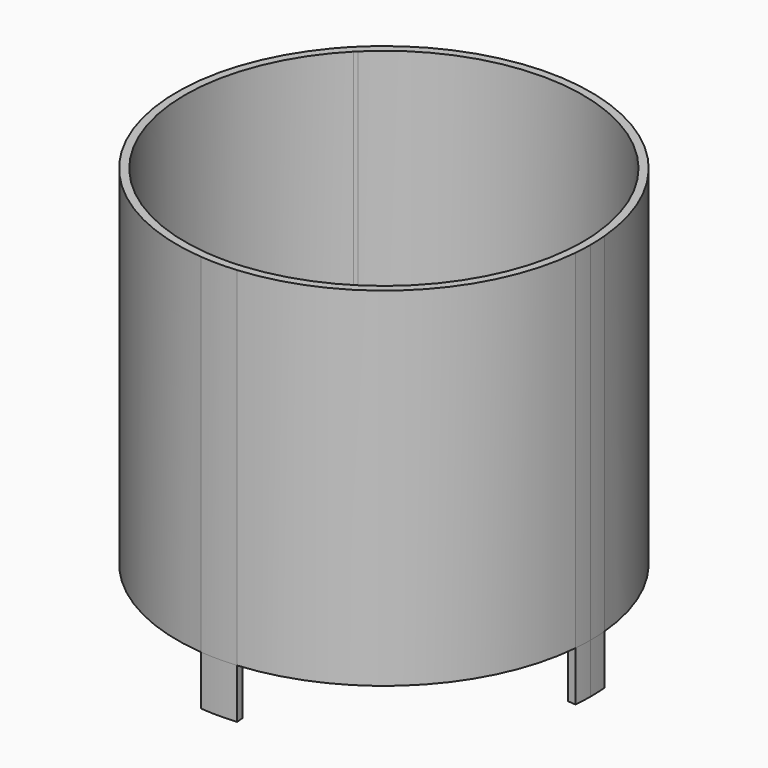
from build123d import *

# Parameters (mm, degrees)
F1_DEPTH = 80
F2_DEPTH = 70


with BuildPart() as f1:
    # F0 (on Top) → F1 (new body)
    with BuildSketch(Plane.XY):
        with BuildLine():
            Line((-70.6127849928, 75.5430583301), (-71.6412451683, 76.7687294391))
            ThreePointArc((-71.6412451683, 76.7687294391), (-74.3169227027, 74.3169227027), (-76.7687294391, 71.6412451683))
            Line((-76.7687294391, 71.6412451683), (-75.5430583301, 70.6127849928))
            ThreePointArc((-75.5430583301, 70.6127849928), (-73.1855518528, 73.1855518528), (-70.6127849928, 75.5430583301))
        make_face()
    extrude(amount=-F1_DEPTH)


with BuildPart() as f1b:
    # F0 (on Top) → F1, piece 2 (new body)
    with BuildSketch(Plane.XY):
        with BuildLine():
            Line((-5.0534926817, 41.4150508954), (-3.4595811647, 41.275601707))
            ThreePointArc((-3.4595811647, 41.275601707), (-3.3408745875, 43.0867140909), (-3.3012806053, 44.9012806053))
            ThreePointArc((-3.3012806053, 44.9012806053), (-3.3408745875, 46.7158471197), (-3.4595811647, 48.5269595036))
            Line((-3.4595811647, 48.5269595036), (-5.0534926817, 48.3875103153))
            ThreePointArc((-5.0534926817, 48.3875103153), (-4.9393517421, 46.6460561), (-4.9012806053, 44.9012806053))
            ThreePointArc((-4.9012806053, 44.9012806053), (-4.9393517421, 43.1565051107), (-5.0534926817, 41.4150508954))
        make_face()
    extrude(amount=-F1_DEPTH)


with BuildPart() as f1c:
    # F0 (on Top) → F1, piece 3 (new body)
    with BuildSketch(Plane.XY):
        with BuildLine():
            ThreePointArc((-48.5269595036, 3.4595811647), (-44.9012806053, 3.3012806053), (-41.275601707, 3.4595811647))
            Line((-41.275601707, 3.4595811647), (-41.4150508954, 5.0534926817))
            ThreePointArc((-41.4150508954, 5.0534926817), (-44.9012806053, 4.9012806053), (-48.3875103153, 5.0534926817))
            Line((-48.3875103153, 5.0534926817), (-48.5269595036, 3.4595811647))
        make_face()
    extrude(amount=-F1_DEPTH)


with BuildPart() as f2:
    # F0 (on Top) → F2 (new body)
    with BuildSketch(Plane.XY):
        with BuildLine():
            Line((-5.0534926817, 48.3875103153), (-3.4595811647, 48.5269595036))
            ThreePointArc((-3.4595811647, 48.5269595036), (-28.981649819, 83.3346691578), (-71.6412451683, 76.7687294391))
            Line((-71.6412451683, 76.7687294391), (-70.6127849928, 75.5430583301))
            ThreePointArc((-70.6127849928, 75.5430583301), (-29.5939433107, 81.8564619058), (-5.0534926817, 48.3875103153))
        make_face()
        with BuildLine():
            Line((-70.6127849928, 75.5430583301), (-71.6412451683, 76.7687294391))
            ThreePointArc((-71.6412451683, 76.7687294391), (-74.3169227027, 74.3169227027), (-76.7687294391, 71.6412451683))
            Line((-76.7687294391, 71.6412451683), (-75.5430583301, 70.6127849928))
            ThreePointArc((-75.5430583301, 70.6127849928), (-73.1855518528, 73.1855518528), (-70.6127849928, 75.5430583301))
        make_face()
        with BuildLine():
            ThreePointArc((-76.7687294391, 71.6412451683), (-83.3346691578, 28.981649819), (-48.5269595036, 3.4595811647))
            Line((-48.5269595036, 3.4595811647), (-48.3875103153, 5.0534926817))
            ThreePointArc((-48.3875103153, 5.0534926817), (-81.8564619058, 29.5939433107), (-75.5430583301, 70.6127849928))
            Line((-75.5430583301, 70.6127849928), (-76.7687294391, 71.6412451683))
        make_face()
        with BuildLine():
            ThreePointArc((-48.5269595036, 3.4595811647), (-44.9012806053, 3.3012806053), (-41.275601707, 3.4595811647))
            Line((-41.275601707, 3.4595811647), (-41.4150508954, 5.0534926817))
            ThreePointArc((-41.4150508954, 5.0534926817), (-44.9012806053, 4.9012806053), (-48.3875103153, 5.0534926817))
            Line((-48.3875103153, 5.0534926817), (-48.5269595036, 3.4595811647))
        make_face()
        with BuildLine():
            ThreePointArc((-41.275601707, 3.4595811647), (-15.485638508, 15.485638508), (-3.4595811647, 41.275601707))
            Line((-3.4595811647, 41.275601707), (-5.0534926817, 41.4150508954))
            ThreePointArc((-5.0534926817, 41.4150508954), (-16.6170093579, 16.6170093579), (-41.4150508954, 5.0534926817))
            Line((-41.4150508954, 5.0534926817), (-41.275601707, 3.4595811647))
        make_face()
        with BuildLine():
            Line((-5.0534926817, 41.4150508954), (-3.4595811647, 41.275601707))
            ThreePointArc((-3.4595811647, 41.275601707), (-3.3408745875, 43.0867140909), (-3.3012806053, 44.9012806053))
            ThreePointArc((-3.3012806053, 44.9012806053), (-3.3408745875, 46.7158471197), (-3.4595811647, 48.5269595036))
            Line((-3.4595811647, 48.5269595036), (-5.0534926817, 48.3875103153))
            ThreePointArc((-5.0534926817, 48.3875103153), (-4.9393517421, 46.6460561), (-4.9012806053, 44.9012806053))
            ThreePointArc((-4.9012806053, 44.9012806053), (-4.9393517421, 43.1565051107), (-5.0534926817, 41.4150508954))
        make_face()
    extrude(amount=-F2_DEPTH)


solid = Compound([f1.part, f1b.part, f1c.part, f2.part])
